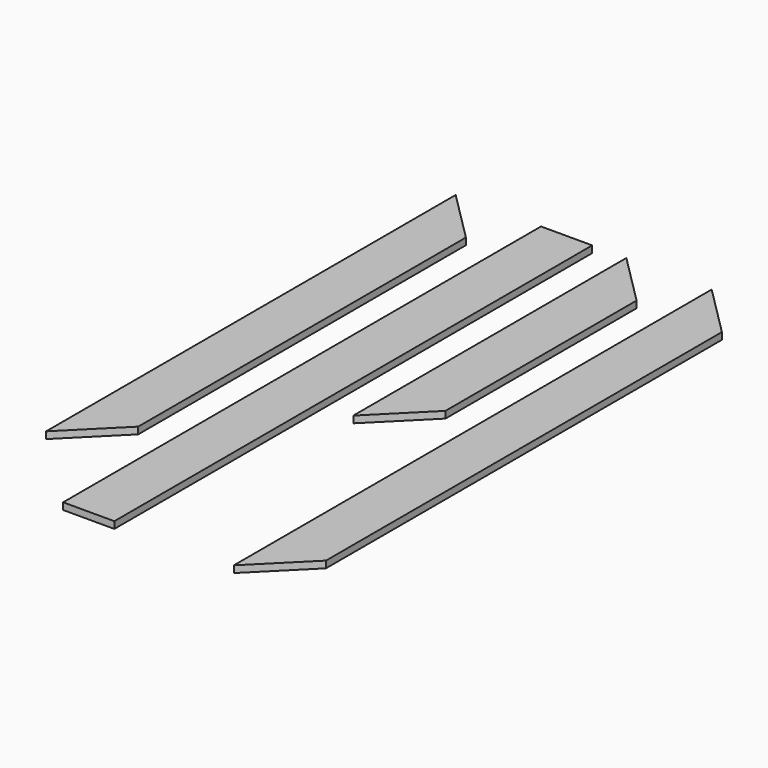
from build123d import *

# Parameters (mm, degrees)
F0_W     = 120
F0_H     = 16
F1_DEPTH = 800
F2_DEPTH = 1200
F4_SIZE  = 119.99999
F6_SIZE  = 119.99999
F7_DEPTH = 1400
F9_SIZE  = 119.99999


# Not quite as in the source:
# - a fillet or chamfer is up to 0.001 mm smaller than in the source, because OpenCascade refuses the exact size


with BuildPart() as f1:
    # F0 (on Front) → F1 (new body)
    with BuildSketch(Plane.XZ):
        Rectangle(F0_W, F0_H)
    extrude(amount=F1_DEPTH)


with BuildPart() as f2:
    # F0 (on Front) → F2 (new body)
    with BuildSketch(Plane.XZ):
        Rectangle(F0_W, F0_H)
    extrude(amount=F2_DEPTH)


with BuildPart() as f3_1:
    # F3: copy of F1
    add(f1.part.moved(Location((200, 0, 0))))

    # F4 (size 120 in the source; OpenCascade refuses exactly that, so slightly less here)
    f4_edges = [f3_1.edges().sort_by_distance(p)[0] for p in [
        (260, -800, 0),
        (260, 0, 0),
    ]]
    chamfer(f4_edges, length=F4_SIZE)


with BuildPart() as f5_1:
    # F5: copy of F2
    add(f2.part.moved(Location((-200, 0, 0))))

    # F6 (size 120 in the source; OpenCascade refuses exactly that, so slightly less here)
    f6_edges = [f5_1.edges().sort_by_distance(p)[0] for p in [
        (-140, -1200, 0),
        (-140, 0, 0),
    ]]
    chamfer(f6_edges, length=F6_SIZE)


with BuildPart() as f7:
    # F0 (on Front) → F7 (new body)
    with BuildSketch(Plane.XZ):
        Rectangle(F0_W, F0_H)
    extrude(amount=F7_DEPTH)


with BuildPart() as f8_1:
    # F8: copy of F7
    add(f7.part.moved(Location((400, 0, 0))))

    # F9 (size 120 in the source; OpenCascade refuses exactly that, so slightly less here)
    f9_edges = [f8_1.edges().sort_by_distance(p)[0] for p in [
        (460, -1400, 0),
        (460, 0, 0),
    ]]
    chamfer(f9_edges, length=F9_SIZE)


solid = Compound([f1.part, f2.part, f3_1.part, f5_1.part, f7.part, f8_1.part])
